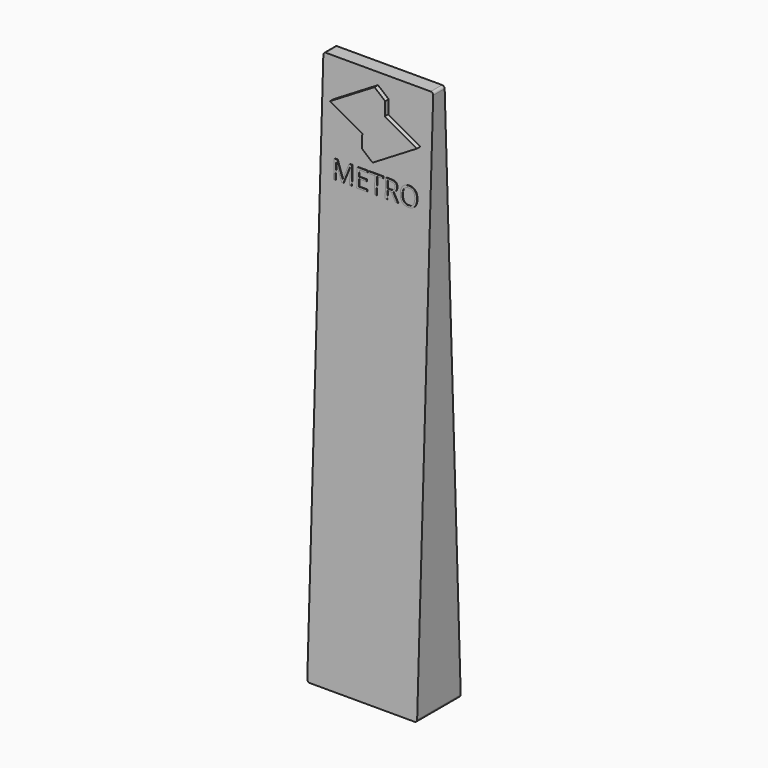
from build123d import *

# Parameters (mm, degrees)
F0_W          = 1000
F0_H          = 5000
F1_DEPTH      = 250
F3_DEPTH      = 1000.001
F4_R          = 20
F6_DEPTH      = 250
F8_DEPTH      = 2500
F10_DEPTH     = 800
F12_DEPTH     = 1003.001
F13_TEXT_SIZE = 234.400036625
F16_DEPTH     = 1003.001


# Not quite as in the source:
# - Text() gives the source's letters only with a copy of the font that has no kerning and outlines rounded to 1/6400 em; it was checked with that copy


with BuildPart() as f1:
    # F0 (on Front) → F1 (new body, symmetric)
    with BuildSketch(Plane.XZ):
        Rectangle(F0_W, F0_H)
    extrude(amount=F1_DEPTH, both=True)

    # F2 (on face) → F3 (cut, through all)
    with BuildSketch(Plane.YZ.offset(500)):
        Polygon((-250, 2500), (-250, -2500), (-62.78, 2560), (-250, 2560), align=None)
        Polygon((250, -2500), (250, 2500), (250, 2560), (62.78, 2560), align=None)
    extrude(amount=-F3_DEPTH, mode=Mode.SUBTRACT)

    # F4
    f4_edges = [f1.edges().sort_by_distance(p)[0] for p in [
        (-500, 0, 2500),
        (500, 0, 2500),
        (-500, 0, -2500),
        (500, 0, -2500),
    ]]
    fillet(f4_edges, radius=F4_R)


with BuildPart() as f6:
    # F5 (on Front) → F6 (new body, symmetric)
    with BuildSketch(Plane.XZ):
        with BuildLine():
            ThreePointArc((-480, 2503), (-496.2634559673, 2496.2634559673), (-503, 2480))
            Line((-503, 2480), (-503, -2480))
            ThreePointArc((-503, -2480), (-496.2634559673, -2496.2634559673), (-480, -2503))
            Line((-480, -2503), (480, -2503))
            ThreePointArc((480, -2503), (496.2634559673, -2496.2634559673), (503, -2480))
            Line((503, -2480), (503, 2480))
            ThreePointArc((503, 2480), (496.2634559673, 2496.2634559673), (480, 2503))
            Line((480, 2503), (-480, 2503))
        make_face()
        with BuildLine():
            ThreePointArc((500, -2480), (494.1421356237, -2494.1421356237), (480, -2500))
            Line((480, -2500), (-480, -2500))
            ThreePointArc((-480, -2500), (-494.1421356237, -2494.1421356237), (-500, -2480))
            Line((-500, -2480), (-500, 2480))
            ThreePointArc((-500, 2480), (-494.1421356237, 2494.1421356237), (-480, 2500))
            Line((-480, 2500), (480, 2500))
            ThreePointArc((480, 2500), (494.1421356237, 2494.1421356237), (500, 2480))
            Line((500, 2480), (500, -2480))
        make_face(mode=Mode.SUBTRACT)
    extrude(amount=F6_DEPTH, both=True)

    # F2 (on face) → F8 (cut, symmetric)
    with BuildSketch(Plane.YZ.offset(500)):
        Polygon((-250, 2500), (-250, -2500), (-62.78, 2560), (-250, 2560), align=None)
        Polygon((250, -2500), (250, 2500), (250, 2560), (62.78, 2560), align=None)
    extrude(amount=F8_DEPTH, both=True, mode=Mode.SUBTRACT)


with BuildPart() as f10:
    # F9 (on offset) → F10 (new body)
    with BuildSketch(Plane.XZ.offset(730)):
        Polygon((100, 2200), (100, 2320), (0, 2400), (-400, 2160), (-100, 2000), (-100, 1880), (0, 1800), (400, 2040), align=None)
    extrude(amount=-F10_DEPTH)

    # F11 (on face) → F12 (cut, through all)
    with BuildSketch(Plane.YZ.offset(500)):
        Polygon((-840.5044209141, 2445.0669842596), (-289.5744301807, -2487.7583660833), (-106.0544301807, 2472.2416339167), align=None)
        Polygon((918.9364817108, 2448.4317301767), (65.74, 2480), (0, 2371.4685440063), (165.3292164933, -2096.8886585164), (249.26, -2480), align=None)
    extrude(amount=-F12_DEPTH, mode=Mode.SUBTRACT)


with BuildPart() as f14:
    # F13 (on offset) → F14 (new body, up to the next surface of F1)
    with BuildSketch(Plane.XZ.offset(730)):
        with Locations((-399.9158390843, 1531.23197363)):
            Text('METRO', F13_TEXT_SIZE, font='Open Sans', text_align=(TextAlign.LEFT, TextAlign.BOTTOM))
    extrude(until=Until.NEXT, target=f1.part, dir=(0, 1, 0))

    # F15 (on face) → F16 (cut, through all)
    with BuildSketch(Plane.YZ.offset(500)):
        Polygon((-869.9077367783, 1424.3061542511), (-109.8040942857, 1424.3061542511), (-98.9092742626, 1718.760749471), (-869.9077367783, 1736.7771863937), align=None)
    extrude(amount=-F16_DEPTH, mode=Mode.SUBTRACT)


with BuildPart() as f17_1:
    # F17: instance of F10
    add(f10.part.mirror(Plane.XZ))


with BuildPart() as f17_2:
    # F17: instance of F14
    add(f14.part.mirror(Plane.XZ))


with BuildPart() as f18_1:
    # F18: instance of F17_1
    add(f17_1.part.mirror(Plane.YZ))


with BuildPart() as f18_2:
    # F18: instance of F17_2
    add(f17_2.part.mirror(Plane.YZ))


solid = Compound([f1.part, f6.part, f10.part, f14.part, f18_1.part, f18_2.part])
